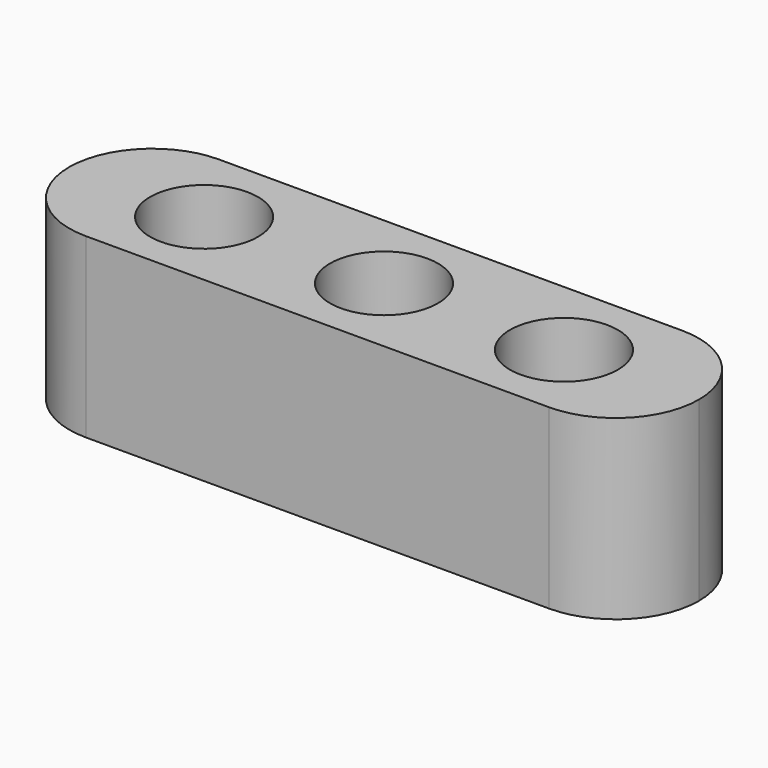
from build123d import *

# Parameters (mm, degrees)
F0_R        = 2.4
F1_DEPTH    = 7.88
F2_T1_DEPTH = 26.405


# Not quite as in the source:
# - a fillet or chamfer that OpenCascade refuses, or shapes differently, is made with other operations: its cross-section is extruded or revolved along the edge and cut away or added


with BuildPart() as f1:
    # F0 (on Top) → F1 (new body)
    with BuildSketch(Plane.XY):
        Polygon((-14.7195083171, 1.6058013724), (-28.7195083171, 1.6058013724), (-42.7195083171, 1.6058013724), (-42.7195083171, -2.0891986276), (-42.7195083171, -5.7841986276), (-28.7195083171, -5.7841986276), (-14.7195083171, -5.7841986276), (-14.7195083171, -2.0891986276), align=None)
        with Locations((-36.7195083171, -2.0891986276)):
            Circle(F0_R, mode=Mode.SUBTRACT)
        with BuildLine():
            ThreePointArc((-28.7195083171, -4.4891986276), (-31.1195083171, -2.0891986276), (-28.7195083171, 0.3108013724))
            ThreePointArc((-28.7195083171, 0.3108013724), (-26.3195083171, -2.0891986276), (-28.7195083171, -4.4891986276))
        make_face(mode=Mode.SUBTRACT)
        with Locations((-20.7195083171, -2.0891986276)):
            Circle(F0_R, mode=Mode.SUBTRACT)
    extrude(amount=F1_DEPTH)

    # F2: fillet of radius 3.705 on 4 edges, made by hand

    # F2_s2 → F2_t1 (cut)
    with BuildSketch(Plane.XY.offset(-9.2625)):
        with BuildLine():
            ThreePointArc((-14.7195083171, -2.0991986276), (-15.8046776928, 0.5206319967), (-18.4245083171, 1.6058013724))
            Line((-18.4245083171, 1.6058013724), (-14.7195083171, 1.6058013724))
            Line((-14.7195083171, 1.6058013724), (-14.7195083171, -2.0991986276))
        make_face()
        with BuildLine():
            ThreePointArc((-14.7195083171, -2.0791986276), (-15.8046776928, -4.6990292519), (-18.4245083171, -5.7841986276))
            Line((-18.4245083171, -5.7841986276), (-14.7195083171, -5.7841986276))
            Line((-14.7195083171, -5.7841986276), (-14.7195083171, -2.0791986276))
        make_face()
        with BuildLine():
            ThreePointArc((-42.7195083171, -2.0991986276), (-41.6343389413, 0.5206319967), (-39.0145083171, 1.6058013724))
            Line((-39.0145083171, 1.6058013724), (-42.7195083171, 1.6058013724))
            Line((-42.7195083171, 1.6058013724), (-42.7195083171, -2.0991986276))
        make_face()
        with BuildLine():
            ThreePointArc((-42.7195083171, -2.0791986276), (-41.6343389413, -4.6990292519), (-39.0145083171, -5.7841986276))
            Line((-39.0145083171, -5.7841986276), (-42.7195083171, -5.7841986276))
            Line((-42.7195083171, -5.7841986276), (-42.7195083171, -2.0791986276))
        make_face()
    extrude(amount=F2_T1_DEPTH, mode=Mode.SUBTRACT)


solid = f1.part
